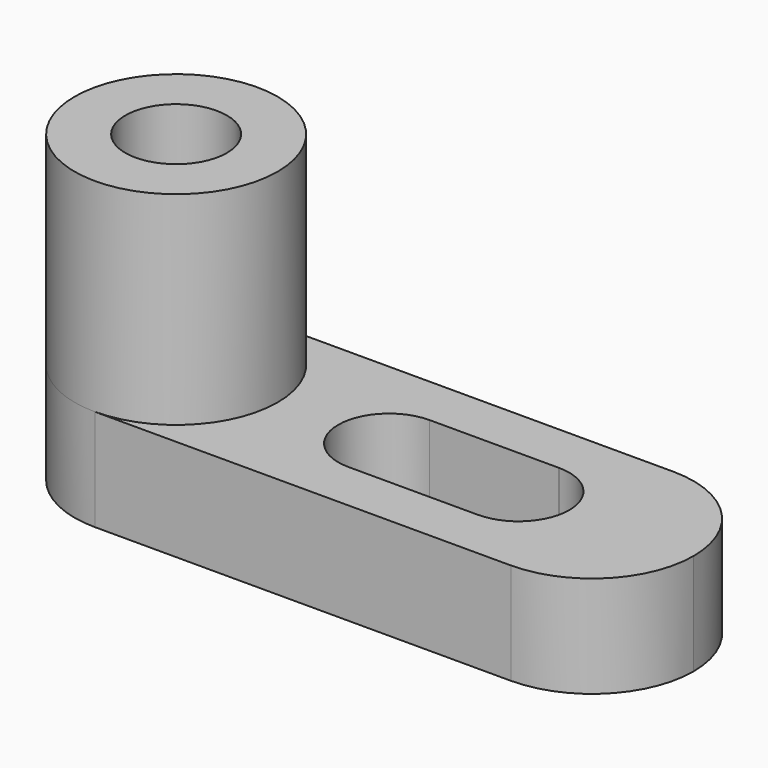
from build123d import *

# Parameters (mm, degrees)
F0_W      = 76.2
F0_H      = 12.7
F1_DEPTH  = 25.4
F3_DEPTH  = 12.7
F5_DEPTH  = 25.4
F6_R      = 6.35
F7_DEPTH  = 25.4
F9_DEPTH  = 25.4
F10_R     = 12.7
F11_DEPTH = 38.1
F12_R     = 6.35
F13_DEPTH = 25.4


with BuildPart() as f1:
    # F0 (on Front) → F1 (new body)
    with BuildSketch(Plane.XZ):
        with Locations((38.1, 6.35)):
            Rectangle(F0_W, F0_H)
    extrude(amount=F1_DEPTH)

    # F2 (on face) → F3 (cut)
    with BuildSketch(Plane.XY.offset(12.7)):
        with BuildLine():
            ThreePointArc((0, -7.291528), (4.686299, -1.976717), (11.490798, 0))
            Line((11.490798, 0), (0, 0))
            Line((0, 0), (0, -7.291528))
        make_face()
        with BuildLine():
            Line((0, -25.4), (11.490798, -25.4))
            ThreePointArc((11.490798, -25.4), (4.686299, -23.423283), (0, -18.108472))
            Line((0, -18.108472), (0, -25.4))
        make_face()
    extrude(amount=-F3_DEPTH, mode=Mode.SUBTRACT)

    # F4 (on face) → F5 (join)
    with BuildSketch(Plane.XY.offset(12.7)):
        with BuildLine():
            Line((0, -18.108472), (0, -7.291528))
            ThreePointArc((0, -7.291528), (-1.209202, -12.7), (0, -18.108472))
        make_face()
    extrude(amount=F5_DEPTH)

    # F6 (on face) → F7 (cut)
    with BuildSketch(Plane.XY.offset(38.1)):
        with Locations((11.490798, -12.7)):
            Circle(F6_R)
    extrude(amount=-F7_DEPTH, mode=Mode.SUBTRACT)

    # F8 (on face) → F9 (cut)
    with BuildSketch(Plane.XY.offset(12.7)):
        with BuildLine():
            ThreePointArc((38.117161, -19.05), (42.607185, -17.190071), (44.467, -12.7))
            ThreePointArc((44.467, -12.7), (42.607185, -8.209929), (38.117161, -6.35))
            ThreePointArc((38.117161, -6.35), (31.767, -12.7), (38.117161, -19.05))
        make_face()
        with BuildLine():
            ThreePointArc((38.117161, -6.35), (42.607185, -8.209929), (44.467, -12.7))
            ThreePointArc((44.467, -12.7), (42.607185, -17.190071), (38.117161, -19.05))
            Line((38.117161, -19.05), (54.299257, -19.05))
            ThreePointArc((54.299257, -19.05), (47.949359, -12.73599), (54.227279, -6.350408))
            Line((54.227279, -6.350408), (38.117161, -6.35))
        make_face()
        with BuildLine():
            Line((54.371558, -6.350412), (54.227279, -6.350408))
            ThreePointArc((54.227279, -6.350408), (47.949359, -12.73599), (54.299257, -19.05))
            ThreePointArc((54.299257, -19.05), (58.789385, -17.190128), (60.649257, -12.7))
            ThreePointArc((60.649257, -12.7), (58.814875, -8.235507), (54.371558, -6.350412))
        make_face()
        with BuildLine():
            ThreePointArc((63.5, 0), (72.480256, -3.719744), (76.2, -12.7))
            Line((76.2, -12.7), (76.2, 0))
            Line((76.2, 0), (63.5, 0))
        make_face()
        with BuildLine():
            ThreePointArc((76.2, -12.7), (72.480256, -21.680256), (63.5, -25.4))
            Line((63.5, -25.4), (76.2, -25.4))
            Line((76.2, -25.4), (76.2, -12.7))
        make_face()
    extrude(amount=-F9_DEPTH, mode=Mode.SUBTRACT)

    # F10 (on face) → F11 (join)
    with BuildSketch(Plane.XY.offset(38.1)):
        with Locations((11.490798, -12.7)):
            Circle(F10_R)
    extrude(amount=-F11_DEPTH)

    # F12 (on face) → F13 (cut)
    with BuildSketch(Plane.XY.offset(38.1)):
        with Locations((11.490798, -12.7)):
            Circle(F12_R)
    extrude(amount=-F13_DEPTH, mode=Mode.SUBTRACT)


solid = f1.part
